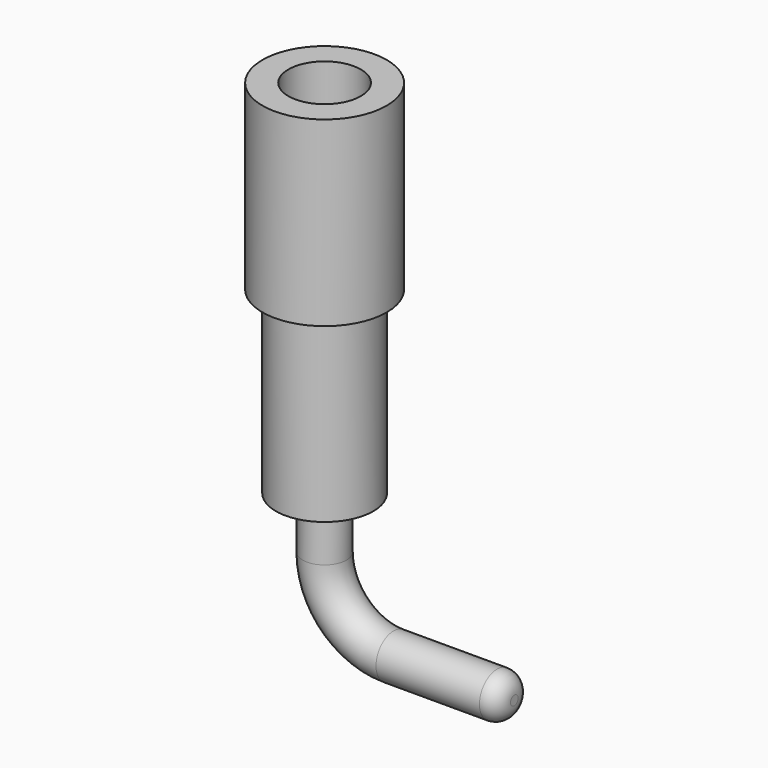
from build123d import *

# Parameters (mm, degrees)
F0_R     = 0.72
F0_R_2   = 0.42
F1_DEPTH = 2.11
F2_R     = 0.565
F2_R_2   = 0.42
F3_DEPTH = 1.57
F4_R     = 0.565
F4_R_2   = 0.42
F5_DEPTH = 0.51
F7_R     = 0.255
F9_R     = 0.2


with BuildPart() as f1:
    # F0 (on Top) → F1 (new body)
    with BuildSketch(Plane.XY):
        Circle(F0_R)
        Circle(F0_R_2, mode=Mode.SUBTRACT)
    extrude(amount=-F1_DEPTH)

    # F2 (on face) → F3 (join)
    with BuildSketch(Plane(origin=(0, 0, -2.11), x_dir=(1, 0, 0), z_dir=(0, 0, -1))):
        Circle(F2_R)
        Circle(F2_R_2, mode=Mode.SUBTRACT)
    extrude(amount=F3_DEPTH)

    # F4 (on face) → F5 (join)
    with BuildSketch(Plane(origin=(0, 0, -3.68), x_dir=(1, 0, 0), z_dir=(0, 0, -1))):
        Circle(F4_R)
        Circle(F4_R_2, mode=Mode.SUBTRACT)
        Circle(F4_R_2)
    extrude(amount=F5_DEPTH)

    # F8: sweep along a path in F6
    with BuildLine(Plane.XZ) as f8_path:
        Line((0, -4.19), (0, -4.79))
        ThreePointArc((0, -4.79), (0.2343145751, -5.3556854249), (0.8, -5.59))
        Line((0.8, -5.59), (2.2, -5.59))
    # F7 (on face) → F8 (sweep)
    with BuildSketch(Plane(origin=(0, 0, -4.19), x_dir=(1, 0, 0), z_dir=(0, 0, -1))):
        Circle(F7_R)
    sweep(path=f8_path.line)

    # F9
    f9_edges = [f1.edges().sort_by_distance(p)[0] for p in [
        (2.2, 0, -5.845),
    ]]
    fillet(f9_edges, radius=F9_R)


solid = f1.part
